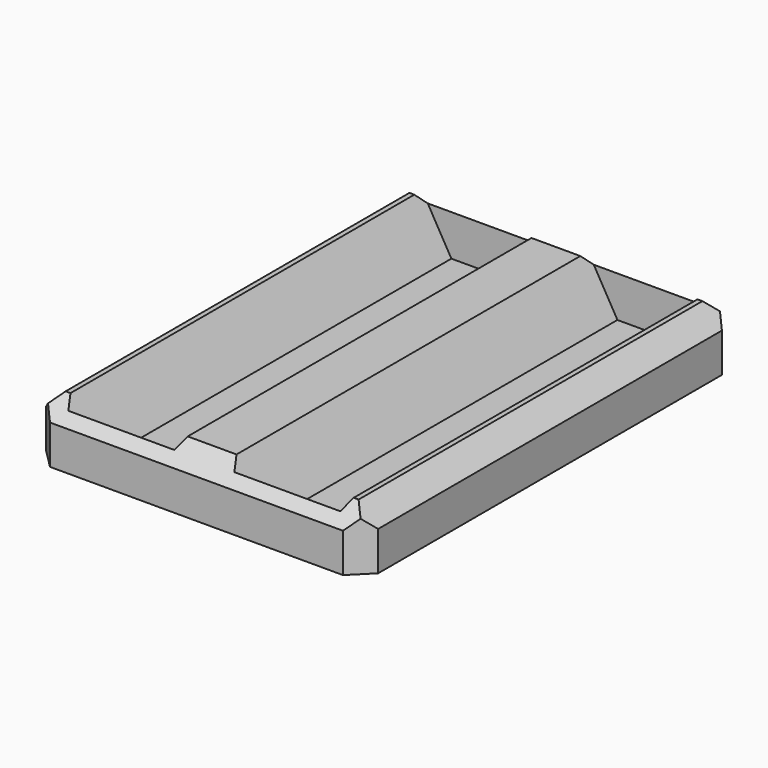
from build123d import *

# Parameters (mm, degrees)
F1_DEPTH    = 116.84
F2_W        = 86.36
F2_H        = 15.24
F3_DEPTH    = 2.54
F4_W        = 86.36
F4_H        = 15.24
F5_DEPTH    = 2.54
F6_T1_DEPTH = 148.0482991577
F6_T3_DEPTH = 112.4882991577
F7_SIZE     = 5.08


# Not quite as in the source:
# - a fillet or chamfer that OpenCascade refuses, or shapes differently, is made with other operations: its cross-section is extruded or revolved along the edge and cut away or added


with BuildPart() as f1:
    # F0 (on Front) → F1 (new body)
    with BuildSketch(Plane.XZ):
        Polygon((43.18, 0), (36.83, 0), (29.21, -13.1982271537), (13.97, -13.1982271537), (6.35, 0), (0, 0), (-6.35, 0), (-13.97, -13.1982271537), (-29.21, -13.1982271537), (-36.83, 0), (-43.18, 0), (-43.18, -15.24), (0, -15.24), (43.18, -15.24), align=None)
    extrude(amount=F1_DEPTH)

    # F2 (on face) → F3 (join)
    with BuildSketch(Plane.XZ.offset(116.84)):
        with Locations((0, -7.62)):
            Rectangle(F2_W, F2_H)
    extrude(amount=F3_DEPTH)

    # F4 (on face) → F5 (join)
    with BuildSketch(Plane(origin=(0, 0, 0), x_dir=(-1, 0, 0), z_dir=(0, 1, 0))):
        with Locations((0, -7.62)):
            Rectangle(F4_W, F4_H)
    extrude(amount=F5_DEPTH)

    # F6: chamfer of 5.08 on 4 edges, made by hand

    # F6_s2 → F6_t1 (cut)
    with BuildSketch(Plane.XZ.offset(-15.6041495789)):
        Polygon((-38.1, 0), (-43.18, -5.08), (-43.18, 0), align=None)
        Polygon((38.1, 0), (43.18, -5.08), (43.18, 0), align=None)
    extrude(amount=F6_T1_DEPTH, mode=Mode.SUBTRACT)

    # F6_s4 → F6_t3 (cut)
    with BuildSketch(Plane.YZ.offset(-56.2441495789)):
        Polygon((-114.3, 0), (-119.38, -5.08), (-119.38, 0), align=None)
        Polygon((-2.54, 0), (2.54, -5.08), (2.54, 0), align=None)
    extrude(amount=F6_T3_DEPTH, mode=Mode.SUBTRACT)

    # F7
    f7_edges = [f1.edges().sort_by_distance(p)[0] for p in [
        (-43.18, -119.38, -10.16),
        (43.18, -119.38, -10.16),
        (43.18, 2.54, -10.16),
        (-43.18, 2.54, -10.16),
    ]]
    chamfer(f7_edges, length=F7_SIZE)


solid = f1.part
